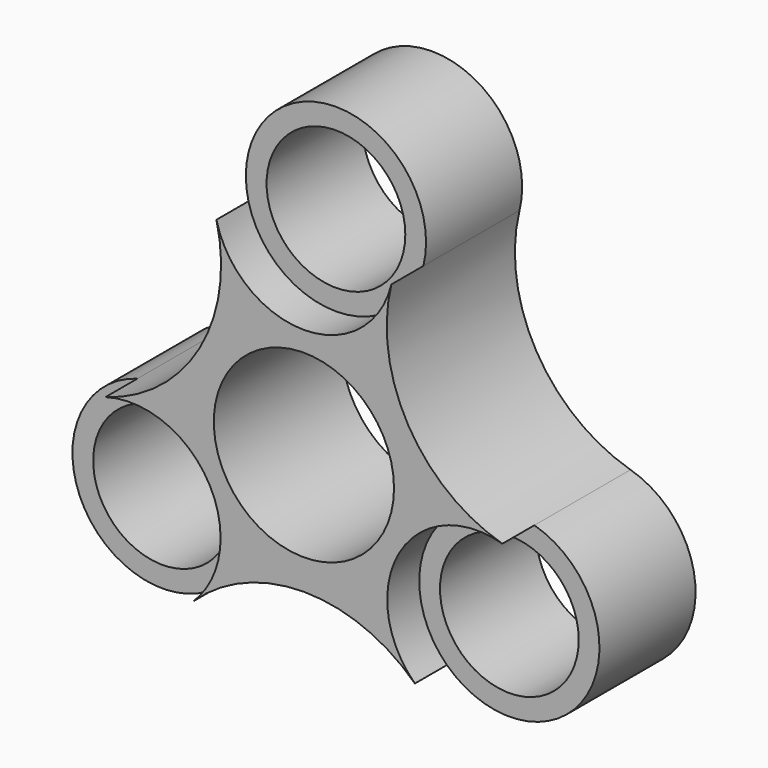
from build123d import *

# Parameters (mm, degrees)
F1_R     = 14.2875
F2_DEPTH = 25.4
F0_R     = 14.2875
F0_R_2   = 10.9982
F3_DEPTH = 19.05


with BuildPart() as f2:
    # F1 (on Front) → F2 (new body)
    with BuildSketch(Plane.XZ):
        with BuildLine():
            ThreePointArc((13.8718760728, 28.3289313848), (0, 17.4625), (-13.8718760728, 28.3289313848))
            ThreePointArc((-13.8718760728, 28.3289313848), (-16.5359438351, 9.5470316245), (-31.4695122777, -2.1510686152))
            ThreePointArc((-31.4695122777, -2.1510686152), (-18.912441482, -4.4535326513), (-13.2088065702, -15.875))
            ThreePointArc((-13.2088065702, -15.875), (-14.3517276668, -21.4743483284), (-17.5976362049, -26.1778627696))
            ThreePointArc((-17.5976362049, -26.1778627696), (0, -19.094063249), (17.5976362049, -26.1778627696))
            ThreePointArc((17.5976362049, -26.1778627696), (15.1229686136, -8.73125), (31.4695122777, -2.1510686152))
            ThreePointArc((31.4695122777, -2.1510686152), (16.5359438351, 9.5470316245), (13.8718760728, 28.3289313848))
        make_face()
        Circle(F1_R, mode=Mode.SUBTRACT)
    extrude(amount=F2_DEPTH)

    # F0 (on Front) → F3 (join)
    with BuildSketch(Plane.XZ):
        with Locations((0, 31.75)):
            Circle(F0_R)
        with Locations((0, 31.75)):
            Circle(F0_R_2, mode=Mode.SUBTRACT)
        with Locations((27.4963065702, -15.875)):
            Circle(F0_R)
        with Locations((27.4963065702, -15.875)):
            Circle(F0_R_2, mode=Mode.SUBTRACT)
        with Locations((-27.4963065702, -15.875)):
            Circle(F0_R)
        with Locations((-27.4963065702, -15.875)):
            Circle(F0_R_2, mode=Mode.SUBTRACT)
    extrude(amount=F3_DEPTH)


solid = f2.part
